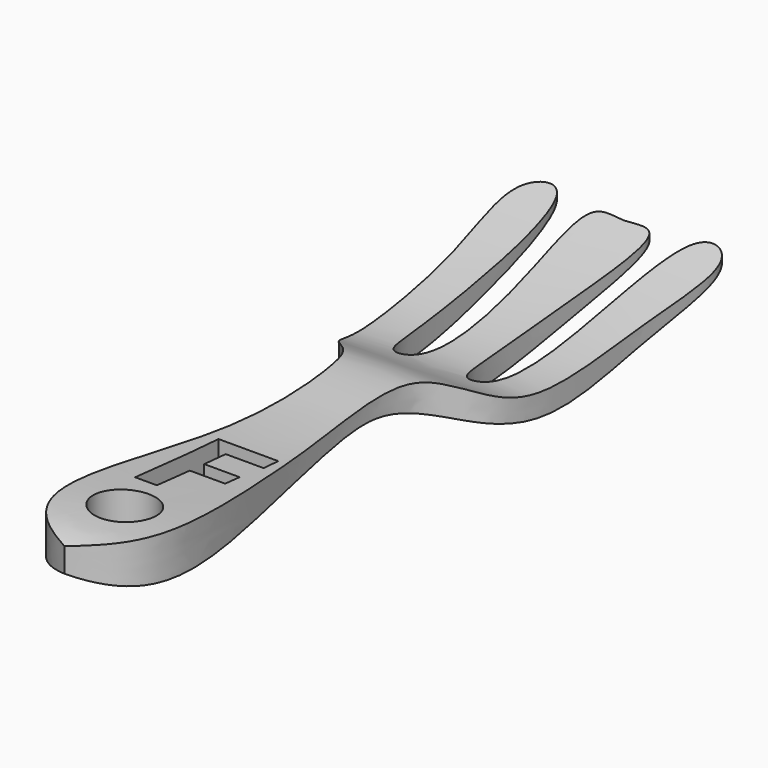
from build123d import *

# Parameters (mm, degrees)
F0_W         = 30
F0_H         = 100
F1_DEPTH     = 30
F3_W         = 100
F3_H         = 30
F4_DEPTH     = 30
F2_W         = 30
F2_H         = 100
F5_DEPTH     = 30
F6_R         = 3.7258790066
F6_TEXT_SIZE = 18.0980242375
F7_DEPTH     = 35


# Not quite as in the source:
# - Text() gives the source's letters only with a copy of the font that has no kerning and outlines rounded to 1/6400 em; it was checked with that copy


with BuildPart() as f1:
    # F0 (on Top) → F1 (new body)
    with BuildSketch(Plane.XY):
        Rectangle(F0_W, F0_H)
    extrude(amount=F1_DEPTH)

    # F3 (on face) → F4 (cut)
    with BuildSketch(Plane.YZ.offset(15)):
        with Locations((0, 15)):
            Rectangle(F3_W, F3_H)
        with BuildLine():
            add(Edge.make_bspline(
                [(45.8902865648, 22.0953244716), (44.7809396176, 22.1410896709), (12.4915015979, 12.5790691998), (4.845797239, 22.0896386486), (-13.2571621319, 17.387543761), (-47.504314909, 23.7937224728), (-46.9398246667, 14.1883031206), (-11.1737781563, 17.2010910698), (-0.716162577, 18.8527038487), (13.5474406355, 12.0068561949), (28.0709291775, 15.5989958497), (46.6875980631, 22.062432039), (45.8902865648, 22.0953244716)],
                knots=[0, 0, 0, 0, 0.133860909, 0.2141317724, 0.317441747, 0.4520377781, 0.4923489703, 0.6298944169, 0.715205452, 0.8022325507, 0.9037912872, 1, 1, 1, 1], degree=3))
        make_face(mode=Mode.SUBTRACT)
    extrude(amount=-F4_DEPTH, mode=Mode.SUBTRACT)

    # F2 (on face) → F5 (cut)
    with BuildSketch(Plane.XY.offset(30)):
        Rectangle(F2_W, F2_H)
        with BuildLine():
            add(Edge.make_bspline(
                [(0, 40.7913662493), (-1.3298656062, 40.877543465), (-5.2288180712, 41.8129780748), (-2.6696468199, 28.5783090896), (-1.7568591123, 10.7443883665), (-8.7338041865, 11.902019373), (-4.6924915876, 44.0175705105), (-14.4837040855, 41.0374992575), (-10.8262271171, 28.3903177645), (-11.7817441359, 7.1517781852), (-1.5259721071, 4.0436864556), (-5.7832339732, -22.8256109928), (-8.2221570936, -39.5317687024), (-3.8563613462, -44.3827333914), (0, -45.8902902901)],
                knots=[0, 0, 0, 0, 0.0449348208, 0.1288667206, 0.2283595072, 0.2662100048, 0.3959628158, 0.4427205058, 0.5276451561, 0.6371922323, 0.7039692049, 0.8257817561, 0.9261479811, 1, 1, 1, 1], degree=3))
            add(Edge.make_bspline(
                [(0, 40.7913662493), (1.3298656062, 40.877543465), (5.2288180712, 41.8129780748), (2.6696468199, 28.5783090896), (1.7568591123, 10.7443883665), (8.7338041865, 11.902019373), (4.6924915876, 44.0175705105), (14.4837040855, 41.0374992575), (10.8262271171, 28.3903177645), (11.7817441359, 7.1517781852), (1.5259721071, 4.0436864556), (5.7832339732, -22.8256109928), (8.2221570936, -39.5317687024), (3.8563613462, -44.3827333914), (0, -45.8902902901)],
                knots=[0, 0, 0, 0, 0.0449348208, 0.1288667206, 0.2283595072, 0.2662100048, 0.3959628158, 0.4427205058, 0.5276451561, 0.6371922323, 0.7039692049, 0.8257817561, 0.9261479811, 1, 1, 1, 1], degree=3))
        make_face(mode=Mode.SUBTRACT)
    extrude(amount=-F5_DEPTH, mode=Mode.SUBTRACT)

    # F6 (on Top) → F7 (cut, symmetric)
    with BuildSketch(Plane.XY):
        with Locations((0, -36.5422666073)):
            Circle(F6_R)
        with Locations((-5.0989221781, -30.5935256183)):
            Text('F', F6_TEXT_SIZE, font='Open Sans', font_style=FontStyle.BOLD, text_align=(TextAlign.LEFT, TextAlign.BOTTOM))
    extrude(amount=F7_DEPTH, both=True, mode=Mode.SUBTRACT)


solid = f1.part
